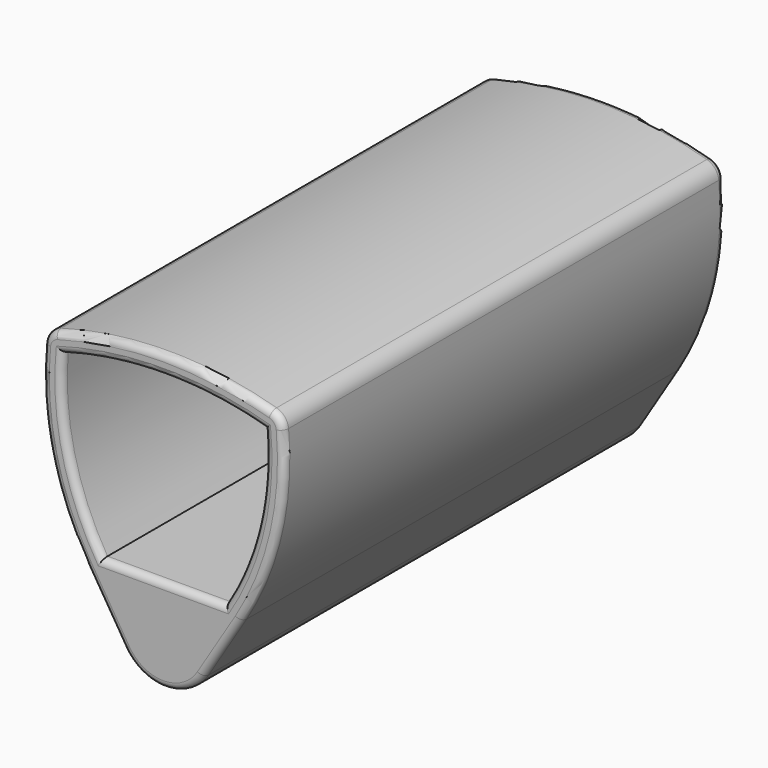
from build123d import *

# Parameters (mm, degrees)
F0_R         = 4.5
F1_DEPTH     = 100
F2_DEPTH     = 3.5
F3_DEPTH     = 100
F4_DEPTH     = 25
F5_R         = 3
F6_T3_ANGLE  = 31.7794665587
F6_T6_ANGLE  = 68.7130750893
F6_T9_ANGLE  = 68.7130750893
F6_T12_ANGLE = 36.7833572648
F6_T15_ANGLE = 36.7833572648
F6_T18_DEPTH = 13.096101665
F6_T21_DEPTH = 13.096101665
F6_T24_ANGLE = 116.6112692326
F6_T27_ANGLE = 36.4778324905
F6_S28_R     = 49.99628125
F6_T29_DEPTH = 26
F6_S30_R     = 49.99628125
F6_T31_DEPTH = 26
F6_T34_ANGLE = 43.5540849409
F6_S35_R     = 67.8625
F6_T36_DEPTH = 23
F6_T40_DEPTH = 28.5
F6_S41_R     = 49.99628125
F6_T42_DEPTH = 16
F6_S43_R     = 49.99628125
F6_T44_DEPTH = 16
F6_T47_ANGLE = 43.5540849409
F6_S48_R     = 67.8625
F6_T49_DEPTH = 23
F6_T54_ANGLE = 36.4778324905
F6_S55_R     = 49.99628125
F6_T56_DEPTH = 26
F6_T59_ANGLE = 43.5540849409
F6_S60_R     = 67.8625
F6_T61_DEPTH = 23
F6_T66_ANGLE = 36.4778324905
F6_S67_R     = 49.99628125
F6_T68_DEPTH = 26
F6_T71_ANGLE = 43.5540849409
F6_S72_R     = 67.8625
F6_T73_DEPTH = 23
F6_T78_ANGLE = 43.5540849409
F6_T82_DEPTH = 28.5
F6_S83_R     = 49.99628125
F6_T84_DEPTH = 16
F6_T89_DEPTH = 28.5
F6_S90_R     = 49.99628125
F6_T91_DEPTH = 16
F6_T94_ANGLE = 43.5540849409
F7_R         = 1.25
F7_R_2       = 1.2499


# Not quite as in the source:
# - a fillet or chamfer that OpenCascade refuses, or shapes differently, is made with other operations: its cross-section is extruded or revolved along the edge and cut away or added
# - a fillet or chamfer is up to 0.001 mm smaller than in the source, because OpenCascade refuses the exact size


with BuildPart() as f1:
    # F0 (on Front) → F1 (new body)
    with BuildSketch(Plane.XZ):
        with BuildLine():
            ThreePointArc((21.473471105, 33.0925985963), (0, 36.4), (-21.473471105, 33.0925985963))
            ThreePointArc((-21.473471105, 33.0925985963), (-20.7900990818, 15.0031031025), (-14.1128680108, -1.8228123189))
            Line((-14.1128680108, -1.8228123189), (-7.2323336433, -12.9657978092))
            ThreePointArc((-7.2323336433, -12.9657978092), (0, -17), (7.2323336433, -12.9657978092))
            Line((7.2323336433, -12.9657978092), (14.1128680108, -1.8228123189))
            ThreePointArc((14.1128680108, -1.8228123189), (20.7900990818, 15.0031031025), (21.473471105, 33.0925985963))
        make_face()
        with Locations((0, -8.5)):
            Circle(F0_R, mode=Mode.SUBTRACT)
        with BuildLine():
            ThreePointArc((18.25, 30.4), (17.1215407764, 14.629521693), (11.125, 0))
            Line((11.125, 0), (-11.125, 0))
            ThreePointArc((-11.125, 0), (-17.1215407764, 14.629521693), (-18.25, 30.4))
            ThreePointArc((-18.25, 30.4), (0, 32.9), (18.25, 30.4))
        make_face(mode=Mode.SUBTRACT)
    extrude(amount=F1_DEPTH)

    # F0 (on Front) → F2 (join)
    with BuildSketch(Plane.XZ):
        with BuildLine():
            Line((-11.125, 0), (11.125, 0))
            ThreePointArc((11.125, 0), (17.1215407764, 14.629521693), (18.25, 30.4))
            ThreePointArc((18.25, 30.4), (0, 32.9), (-18.25, 30.4))
            ThreePointArc((-18.25, 30.4), (-17.1215407764, 14.629521693), (-11.125, 0))
        make_face()
    extrude(amount=F2_DEPTH)

    # F0 (on Front) → F3 (join)
    with BuildSketch(Plane.XZ):
        with Locations((0, -8.5)):
            Circle(F0_R)
    extrude(amount=F3_DEPTH)

    # F0 (on Front) → F4 (cut)
    with BuildSketch(Plane.XZ):
        with Locations((0, -8.5)):
            Circle(F0_R)
    extrude(amount=F4_DEPTH, mode=Mode.SUBTRACT)

    # F5
    f5_edges = [f1.edges().sort_by_distance(p)[0] for p in [
        (-21.473471, -50, 33.092599),
        (21.473471, -50, 33.092599),
    ]]
    fillet(f5_edges, radius=F5_R)

    # F6: fillet of radius 1.25 on 12 edges, made by hand


with BuildPart() as f6_tool1:
    # F6_s2 → F6_t3 (revolve)
    with BuildSketch(Plane(origin=(9.2065209471, 0, -2.6207630089), x_dir=(0, 1, 0), z_dir=(0.9617903843, 0, -0.2737868817))):
        with BuildLine():
            ThreePointArc((-98.75, 37.7359036877), (-99.6338834765, 37.3697871642), (-100, 36.4859036877))
            Line((-100, 36.4859036877), (-100, 37.7359036877))
            Line((-100, 37.7359036877), (-98.75, 37.7359036877))
        make_face()
    revolve(axis=Axis((0, -100, -34.9625), (0, -1, 0)), revolution_arc=F6_T3_ANGLE)


with BuildPart() as f6_tool4:
    # F6_s5 → F6_t6 (revolve)
    with BuildSketch(Plane(origin=(9.2065210076, 0, -2.6207630106), x_dir=(0, 1, 0), z_dir=(-0.9617903848, 0, 0.2737868802))):
        with BuildLine():
            ThreePointArc((-98.75, -37.7359036714), (-99.6338834765, -37.3697871478), (-100, -36.4859036714))
            Line((-100, -36.4859036714), (-100, -37.7359036728))
            Line((-100, -37.7359036728), (-98.75, -37.7359036714))
        make_face()
    revolve(axis=Axis((18.7167557078, -100, 30.7878951544), (0, 1, 0)), revolution_arc=F6_T6_ANGLE)


with BuildPart() as f6_tool7:
    # F6_s8 → F6_t9 (revolve)
    with BuildSketch(Plane(origin=(-9.2065210076, 0, -2.6207630106), x_dir=(0, 1, 0), z_dir=(0.9617903848, 0, 0.2737868802))):
        with BuildLine():
            ThreePointArc((-98.75, 37.7359036714), (-99.6338834765, 37.3697871478), (-100, 36.4859036714))
            Line((-100, 36.4859036714), (-100, 37.7359036728))
            Line((-100, 37.7359036728), (-98.75, 37.7359036714))
        make_face()
    revolve(axis=Axis((-18.7167557078, -100, 30.7878951544), (0, -1, 0)), revolution_arc=F6_T9_ANGLE)


with BuildPart() as f6_tool10:
    # F6_s11 → F6_t12 (revolve)
    with BuildSketch(Plane(origin=(3.0175039055, 0, 4.9461501321), x_dir=(0, 1, 0), z_dir=(-0.5208035197, 0, -0.8536765745))):
        with BuildLine():
            ThreePointArc((-100, 11.7471518916), (-99.6338834765, 12.631035368), (-98.75, 12.9971518916))
            Line((-98.75, 12.9971518916), (-100, 12.9971518916))
            Line((-100, 12.9971518916), (-100, 11.7471518916))
        make_face()
    revolve(axis=Axis((-31.5556541163, -100, 26.038239246), (0, -1, 0)), revolution_arc=F6_T12_ANGLE)


with BuildPart() as f6_tool13:
    # F6_s14 → F6_t15 (revolve)
    with BuildSketch(Plane(origin=(2.7174651154, 0, 28.7628246621), x_dir=(0, 1, 0), z_dir=(0.0940595186, 0, 0.9955665759))):
        with BuildLine():
            ThreePointArc((-100, 23.2796709798), (-99.6338834765, 24.1635544563), (-98.75, 24.5296709798))
            Line((-98.75, 24.5296709798), (-100, 24.5296709798))
            Line((-100, 24.5296709798), (-100, 23.2796709798))
        make_face()
    revolve(axis=Axis((31.5556541163, -100, 26.038239246), (0, -1, 0)), revolution_arc=F6_T15_ANGLE)


with BuildPart() as f6_tool16:
    # F6_s17 → F6_t18 (new body)
    with BuildSketch(Plane(origin=(-3.7997811458, 0, -6.1537235209), x_dir=(0, 1, 0), z_dir=(0.5253879775, 0, 0.8508627816))):
        with BuildLine():
            ThreePointArc((-100, -11.7157978092), (-99.6338834765, -12.5996812857), (-98.75, -12.9657978092))
            Line((-98.75, -12.9657978092), (-100, -12.9657978092))
            Line((-100, -12.9657978092), (-100, -11.7157978092))
        make_face()
    extrude(amount=F6_T18_DEPTH)


with BuildPart() as f6_tool19:
    # F6_s20 → F6_t21 (new body)
    with BuildSketch(Plane(origin=(-3.0807532218, 0, 4.9892619694), x_dir=(0, 1, 0), z_dir=(0.5253879775, 0, -0.8508627816))):
        with BuildLine():
            ThreePointArc((-100, -11.7157978092), (-99.6338834765, -12.5996812857), (-98.75, -12.9657978092))
            Line((-98.75, -12.9657978092), (-100, -12.9657978092))
            Line((-100, -12.9657978092), (-100, -11.7157978092))
        make_face()
    extrude(amount=F6_T21_DEPTH)


with BuildPart() as f6_tool22:
    # F6_s23 → F6_t24 (revolve)
    with BuildSketch(Plane(origin=(3.7997811458, 0, -6.1537235209), x_dir=(0, 1, 0), z_dir=(-0.5253879775, 0, 0.8508627816))):
        with BuildLine():
            ThreePointArc((-100, 11.7157978092), (-99.6338834765, 12.5996812857), (-98.75, 12.9657978092))
            Line((-98.75, 12.9657978092), (-100, 12.9657978092))
            Line((-100, 12.9657978092), (-100, 11.7157978092))
        make_face()
    revolve(axis=Axis((0, -100, -8.5), (0, -1, 0)), revolution_arc=F6_T24_ANGLE)


with BuildPart() as f6_tool25:
    # F6_s26 → F6_t27 (revolve)
    with BuildSketch(Plane(origin=(-10.3928082362, 0, -3.4248052672), x_dir=(0, 1, 0), z_dir=(-0.9497596893, 0, -0.3129800832))):
        with BuildLine():
            ThreePointArc((-100, -35.9065268612), (-99.6338834765, -35.0226433847), (-98.75, -34.6565268612))
            Line((-98.75, -34.6565268612), (-100, -34.6565268612))
            Line((-100, -34.6565268612), (-100, -35.9065268612))
        make_face()
    revolve(axis=Axis((0, -100, -34.9625), (0, 1, 0)), revolution_arc=F6_T27_ANGLE)

    # F6_s28 → F6_t29 (intersect, symmetric)
    with BuildSketch(Plane.XZ.offset(98.9)):
        with Locations((-31.5556541163, 26.038239246)):
            Circle(F6_S28_R)
    extrude(amount=F6_T29_DEPTH, both=True, mode=Mode.INTERSECT)

    # F6_s30 → F6_t31 (intersect, symmetric)
    with BuildSketch(Plane.XZ.offset(98.9)):
        with Locations((31.5556541163, 26.038239246)):
            Circle(F6_S30_R)
    extrude(amount=F6_T31_DEPTH, both=True, mode=Mode.INTERSECT)


with BuildPart() as f6_tool32:
    # F6_s33 → F6_t34 (revolve)
    with BuildSketch(Plane(origin=(-4.5473698948, 0, 30.1163163037), x_dir=(0, 1, 0), z_dir=(-0.1493011914, 0, 0.9887917649))):
        with BuildLine():
            ThreePointArc((-100, -23.9318504655), (-99.6338834765, -23.0479669891), (-98.75, -22.6818504655))
            Line((-98.75, -22.6818504655), (-100, -22.6818504655))
            Line((-100, -22.6818504655), (-100, -23.9318504655))
        make_face()
    revolve(axis=Axis((-31.5556541163, -100, 26.038239246), (0, 1, 0)), revolution_arc=F6_T34_ANGLE)

    # F6_s35 → F6_t36 (intersect, symmetric)
    with BuildSketch(Plane.XZ.offset(98.9)):
        with Locations((0, -34.9625)):
            Circle(F6_S35_R)
    extrude(amount=F6_T36_DEPTH, both=True, mode=Mode.INTERSECT)

    split(bisect_by=Plane.XY, keep=Keep.TOP)


with BuildPart() as f6_tool38:
    # F6_s39 → F6_t40 (new body)
    with BuildSketch(Plane.YZ.offset(14.25)):
        with BuildLine():
            ThreePointArc((-100, -1.25), (-99.6338834765, -0.3661165235), (-98.75, 0))
            Line((-98.75, 0), (-100, 0))
            Line((-100, 0), (-100, -1.25))
        make_face()
    extrude(amount=-F6_T40_DEPTH)

    # F6_s41 → F6_t42 (intersect, symmetric)
    with BuildSketch(Plane.XZ.offset(99.4)):
        with Locations((-31.5556541163, 26.038239246)):
            Circle(F6_S41_R)
    extrude(amount=F6_T42_DEPTH, both=True, mode=Mode.INTERSECT)

    # F6_s43 → F6_t44 (intersect, symmetric)
    with BuildSketch(Plane.XZ.offset(99.4)):
        with Locations((31.5556541163, 26.038239246)):
            Circle(F6_S43_R)
    extrude(amount=F6_T44_DEPTH, both=True, mode=Mode.INTERSECT)


with BuildPart() as f6_tool45:
    # F6_s46 → F6_t47 (revolve)
    with BuildSketch(Plane(origin=(-1.8641799133, 0, 2.6655264084), x_dir=(0, 1, 0), z_dir=(0.5731138857, 0, -0.8194757312))):
        with BuildLine():
            ThreePointArc((-100, -10.4643120484), (-99.6338834765, -9.5804285719), (-98.75, -9.2143120484))
            Line((-98.75, -9.2143120484), (-100, -9.2143120484))
            Line((-100, -9.2143120484), (-100, -10.4643120484))
        make_face()
    revolve(axis=Axis((31.5556541163, -100, 26.038239246), (0, 1, 0)), revolution_arc=F6_T47_ANGLE)

    # F6_s48 → F6_t49 (intersect, symmetric)
    with BuildSketch(Plane.XZ.offset(98.9)):
        with Locations((0, -34.9625)):
            Circle(F6_S48_R)
    extrude(amount=F6_T49_DEPTH, both=True, mode=Mode.INTERSECT)

    split(bisect_by=Plane.XY, keep=Keep.TOP)


with BuildPart() as f6_tool52:
    # F6_s53 → F6_t54 (revolve)
    with BuildSketch(Plane(origin=(-10.3928082362, 0, -3.4248052672), x_dir=(0, 1, 0), z_dir=(-0.9497596893, 0, -0.3129800832))):
        with BuildLine():
            ThreePointArc((-100, -35.9065268612), (-99.6338834765, -35.0226433847), (-98.75, -34.6565268612))
            Line((-98.75, -34.6565268612), (-100, -34.6565268612))
            Line((-100, -34.6565268612), (-100, -35.9065268612))
        make_face()
    revolve(axis=Axis((0, -100, -34.9625), (0, 1, 0)), revolution_arc=F6_T54_ANGLE)

    # F6_s55 → F6_t56 (cut, symmetric)
    with BuildSketch(Plane.XZ.offset(98.9)):
        with Locations((31.5556541163, 26.038239246)):
            Circle(F6_S55_R)
    extrude(amount=F6_T56_DEPTH, both=True, mode=Mode.SUBTRACT)


with BuildPart() as f6_tool57:
    # F6_s58 → F6_t59 (revolve)
    with BuildSketch(Plane(origin=(-1.8641799133, 0, 2.6655264084), x_dir=(0, 1, 0), z_dir=(0.5731138857, 0, -0.8194757312))):
        with BuildLine():
            ThreePointArc((-100, -10.4643120484), (-99.6338834765, -9.5804285719), (-98.75, -9.2143120484))
            Line((-98.75, -9.2143120484), (-100, -9.2143120484))
            Line((-100, -9.2143120484), (-100, -10.4643120484))
        make_face()
    revolve(axis=Axis((31.5556541163, -100, 26.038239246), (0, 1, 0)), revolution_arc=F6_T59_ANGLE)

    # F6_s60 → F6_t61 (cut, symmetric)
    with BuildSketch(Plane.XZ.offset(98.9)):
        with Locations((0, -34.9625)):
            Circle(F6_S60_R)
    extrude(amount=F6_T61_DEPTH, both=True, mode=Mode.SUBTRACT)


with BuildPart() as f6_tool52_1:
    add(f6_tool52.part)

    # F6_t62: intersect F6_tool57
    add(f6_tool57.part, mode=Mode.INTERSECT)


with BuildPart() as f6_tool64:
    # F6_s65 → F6_t66 (revolve)
    with BuildSketch(Plane(origin=(-10.3928082362, 0, -3.4248052672), x_dir=(0, 1, 0), z_dir=(-0.9497596893, 0, -0.3129800832))):
        with BuildLine():
            ThreePointArc((-100, -35.9065268612), (-99.6338834765, -35.0226433847), (-98.75, -34.6565268612))
            Line((-98.75, -34.6565268612), (-100, -34.6565268612))
            Line((-100, -34.6565268612), (-100, -35.9065268612))
        make_face()
    revolve(axis=Axis((0, -100, -34.9625), (0, 1, 0)), revolution_arc=F6_T66_ANGLE)

    # F6_s67 → F6_t68 (cut, symmetric)
    with BuildSketch(Plane.XZ.offset(98.9)):
        with Locations((-31.5556541163, 26.038239246)):
            Circle(F6_S67_R)
    extrude(amount=F6_T68_DEPTH, both=True, mode=Mode.SUBTRACT)


with BuildPart() as f6_tool69:
    # F6_s70 → F6_t71 (revolve)
    with BuildSketch(Plane(origin=(-4.5473698948, 0, 30.1163163037), x_dir=(0, 1, 0), z_dir=(-0.1493011914, 0, 0.9887917649))):
        with BuildLine():
            ThreePointArc((-100, -23.9318504655), (-99.6338834765, -23.0479669891), (-98.75, -22.6818504655))
            Line((-98.75, -22.6818504655), (-100, -22.6818504655))
            Line((-100, -22.6818504655), (-100, -23.9318504655))
        make_face()
    revolve(axis=Axis((-31.5556541163, -100, 26.038239246), (0, 1, 0)), revolution_arc=F6_T71_ANGLE)

    # F6_s72 → F6_t73 (cut, symmetric)
    with BuildSketch(Plane.XZ.offset(98.9)):
        with Locations((0, -34.9625)):
            Circle(F6_S72_R)
    extrude(amount=F6_T73_DEPTH, both=True, mode=Mode.SUBTRACT)


with BuildPart() as f6_tool64_1:
    add(f6_tool64.part)

    # F6_t74: intersect F6_tool69
    add(f6_tool69.part, mode=Mode.INTERSECT)


with BuildPart() as f6_tool76:
    # F6_s77 → F6_t78 (revolve)
    with BuildSketch(Plane(origin=(-4.5473698948, 0, 30.1163163037), x_dir=(0, 1, 0), z_dir=(-0.1493011914, 0, 0.9887917649))):
        with BuildLine():
            ThreePointArc((-100, -23.9318504655), (-99.6338834765, -23.0479669891), (-98.75, -22.6818504655))
            Line((-98.75, -22.6818504655), (-100, -22.6818504655))
            Line((-100, -22.6818504655), (-100, -23.9318504655))
        make_face()
    revolve(axis=Axis((-31.5556541163, -100, 26.038239246), (0, 1, 0)), revolution_arc=F6_T78_ANGLE)

    split(bisect_by=Plane.XY, keep=Keep.BOTTOM)


with BuildPart() as f6_tool80:
    # F6_s81 → F6_t82 (new body)
    with BuildSketch(Plane.YZ.offset(14.25)):
        with BuildLine():
            ThreePointArc((-100, -1.25), (-99.6338834765, -0.3661165235), (-98.75, 0))
            Line((-98.75, 0), (-100, 0))
            Line((-100, 0), (-100, -1.25))
        make_face()
    extrude(amount=-F6_T82_DEPTH)

    # F6_s83 → F6_t84 (cut, symmetric)
    with BuildSketch(Plane.XZ.offset(99.4)):
        with Locations((-31.5556541163, 26.038239246)):
            Circle(F6_S83_R)
    extrude(amount=F6_T84_DEPTH, both=True, mode=Mode.SUBTRACT)


with BuildPart() as f6_tool76_1:
    add(f6_tool76.part)

    # F6_t85: intersect F6_tool80
    add(f6_tool80.part, mode=Mode.INTERSECT)


with BuildPart() as f6_tool87:
    # F6_s88 → F6_t89 (new body)
    with BuildSketch(Plane.YZ.offset(14.25)):
        with BuildLine():
            ThreePointArc((-100, -1.25), (-99.6338834765, -0.3661165235), (-98.75, 0))
            Line((-98.75, 0), (-100, 0))
            Line((-100, 0), (-100, -1.25))
        make_face()
    extrude(amount=-F6_T89_DEPTH)

    # F6_s90 → F6_t91 (cut, symmetric)
    with BuildSketch(Plane.XZ.offset(99.4)):
        with Locations((31.5556541163, 26.038239246)):
            Circle(F6_S90_R)
    extrude(amount=F6_T91_DEPTH, both=True, mode=Mode.SUBTRACT)


with BuildPart() as f6_tool92:
    # F6_s93 → F6_t94 (revolve)
    with BuildSketch(Plane(origin=(-1.8641799133, 0, 2.6655264084), x_dir=(0, 1, 0), z_dir=(0.5731138857, 0, -0.8194757312))):
        with BuildLine():
            ThreePointArc((-100, -10.4643120484), (-99.6338834765, -9.5804285719), (-98.75, -9.2143120484))
            Line((-98.75, -9.2143120484), (-100, -9.2143120484))
            Line((-100, -9.2143120484), (-100, -10.4643120484))
        make_face()
    revolve(axis=Axis((31.5556541163, -100, 26.038239246), (0, 1, 0)), revolution_arc=F6_T94_ANGLE)

    split(bisect_by=Plane.XY, keep=Keep.BOTTOM)


with BuildPart() as f6_tool87_1:
    add(f6_tool87.part)

    # F6_t96: intersect F6_tool92
    add(f6_tool92.part, mode=Mode.INTERSECT)


with BuildPart() as f1_1:
    add(f1.part)

    # F6_t97: cut F6_tool1, F6_tool4, F6_tool7, F6_tool10, F6_tool13, F6_tool16, F6_tool19, F6_tool22, F6_tool25, F6_tool32, F6_tool38, F6_tool45, F6_tool52, F6_tool64, F6_tool76, F6_tool87
    add([f6_tool1.part, f6_tool4.part, f6_tool7.part, f6_tool10.part, f6_tool13.part, f6_tool16.part, f6_tool19.part, f6_tool22.part, f6_tool25.part, f6_tool32.part, f6_tool38.part, f6_tool45.part, f6_tool52_1.part, f6_tool64_1.part, f6_tool76_1.part, f6_tool87_1.part], mode=Mode.SUBTRACT)

    # F7 (call 1 of 4: OpenCascade refuses the feature's edges together)
    f7_edges = [f1_1.edges().sort_by_distance(p)[0] for p in [
        (0, 0, 36.4),
        (21.023156, 0, 32.706362),
        (-21.023156, 0, 32.706362),
        (20.570679, 0, 14.00921),
        (-20.570679, 0, 14.00921),
        (10.672601, 0, -7.394305),
        (-10.672601, 0, -7.394305),
        (0, 0, -17),
    ]]
    fillet(f7_edges, radius=F7_R)

    # F7#2 (call 2 of 4)
    f7_2_edges = [f1_1.edges().sort_by_distance(p)[0] for p in [
        (-4.5, 0, -8.5),
    ]]
    fillet(f7_2_edges, radius=F7_R)

    # F7#3 (call 3 of 4) (radius 1.25 in the source; OpenCascade refuses exactly that, so slightly less here)
    f7_3_edges = [f1_1.edges().sort_by_distance(p)[0] for p in [
        (-10.672601, -100, -7.394305),
    ]]
    fillet(f7_3_edges, radius=F7_R_2)

    # F7#4 (call 4 of 4) (radius 1.25 in the source; OpenCascade refuses exactly that, so slightly less here)
    f7_4_edges = [f1_1.edges().sort_by_distance(p)[0] for p in [
        (10.672601, -100, -7.394305),
    ]]
    fillet(f7_4_edges, radius=F7_R_2)


solid = f1_1.part
